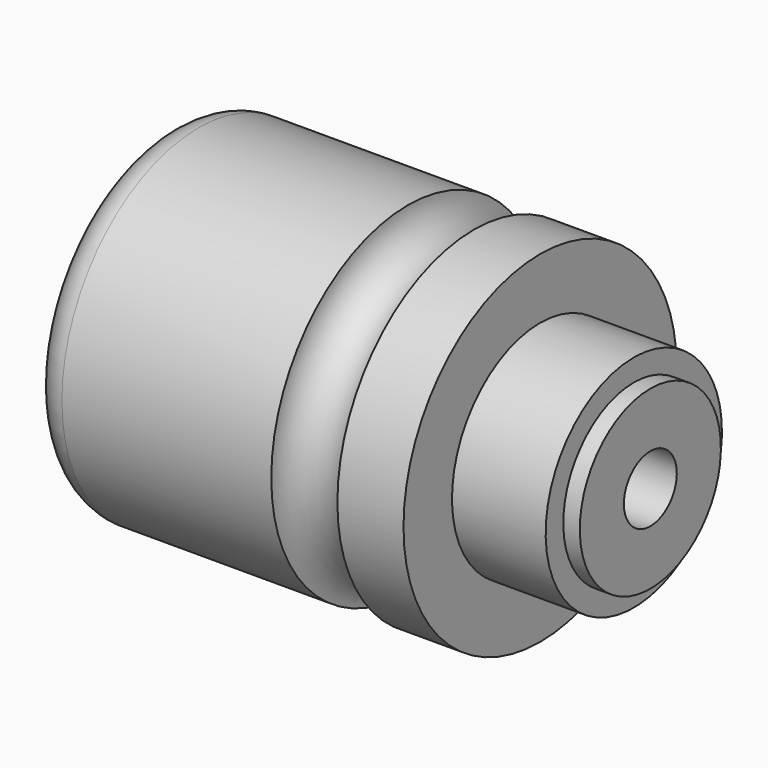
from build123d import *

# Parameters (mm, degrees)
F4_R = 5.99999


# Not quite as in the source:
# - a fillet or chamfer is up to 0.001 mm smaller than in the source, because OpenCascade refuses the exact size


with BuildPart() as f1:
    # F0 (on Front) → F1 (revolve)
    with BuildSketch(Plane.XZ):
        with BuildLine():
            Line((0, 31), (0, 0))
            Line((0, 0), (88, 0))
            Line((88, 0), (88, 16))
            Line((88, 16), (85, 16))
            Line((85, 16), (85, 20))
            Line((85, 20), (68, 20))
            Line((68, 20), (68, 31))
            Line((68, 31), (56, 31))
            ThreePointArc((56, 31), (50, 25), (44, 31))
            Line((44, 31), (0, 31))
        make_face()
    revolve(axis=Axis((55.2076362073, 0, 0), (1, 0, 0)))

    # F2 (on Front) → F3 (revolve, cut)
    with BuildSketch(Plane.XZ):
        Polygon((0, 25), (0, 0), (88, 0), (88, 6), (30, 6), (30, 16), (22, 16), (22, 20.5), (15, 20.5), (15, 12.5), (12, 12.5), (12, 16), (1.5, 16), (1.5, 25), align=None)
    revolve(axis=Axis((-14.1267481727, 0, 0), (-1, 0, 0)), mode=Mode.SUBTRACT)

    # F4 (radius 6 in the source; OpenCascade refuses exactly that, so slightly less here)
    f4_edges = [f1.edges().sort_by_distance(p)[0] for p in [
        (0, 0, -31),
    ]]
    fillet(f4_edges, radius=F4_R)


solid = f1.part
